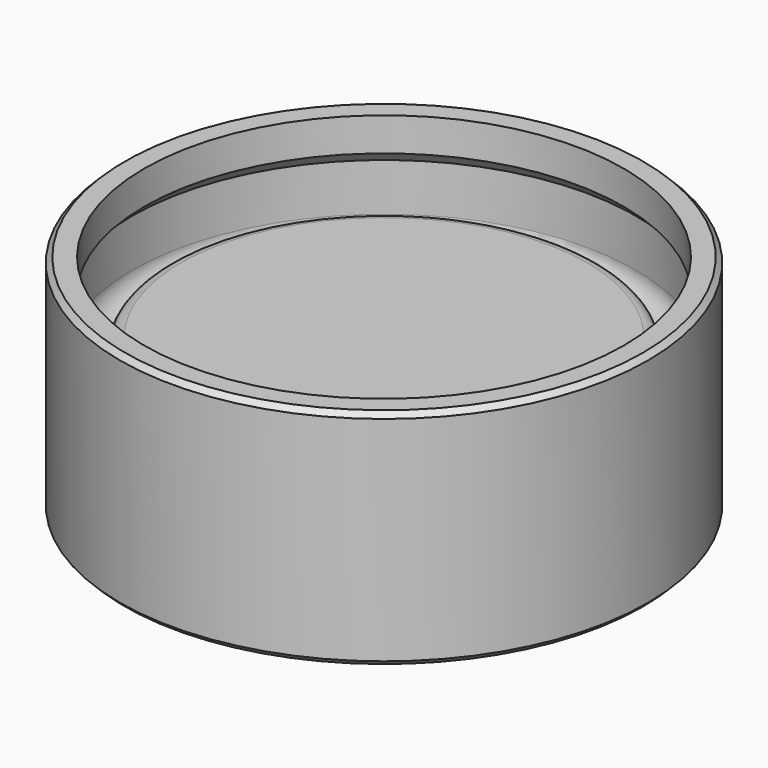
from build123d import *

# Parameters (mm, degrees)
F0_R            = 26
F1_DEPTH        = 22
F2_W            = 8.4
F2_H            = 2.4
F3_DEPTH        = 10
F3_COPIES_COUNT = 14
F4_R            = 4
F5_R            = 20
F6_DEPTH        = 13
F7_R            = 7.9
F8_DEPTH        = 1
F9_R            = 4.75
F10_DEPTH       = 0.8
F11_R           = 23.6
F12_DEPTH       = 7
F13_R           = 24.8
F13_R_2         = 21.2
F14_DEPTH       = 4
F14_DEPTH_BACK  = 4
F15_R           = 1.79999
F16_R           = 1.2
F17_S5_R        = 23.6
F17_T6_DEPTH    = 37
F18_R           = 1
F19_SIZE        = 0.5
F20_R           = 24.3
F21_DEPTH       = 1.5


# Not quite as in the source:
# - a fillet or chamfer that OpenCascade refuses, or shapes differently, is made with other operations: its cross-section is extruded or revolved along the edge and cut away or added
# - a fillet or chamfer is up to 0.001 mm smaller than in the source, because OpenCascade refuses the exact size
# - a pattern or mirror of a feature is missing from the dataset's text; its kind, count and spacing are read off the source's solid


with BuildPart() as f1:
    # F0 (on Top) → F1 (new body)
    with BuildSketch(Plane.XY):
        Circle(F0_R)
    extrude(amount=F1_DEPTH)

    # F2 (on face) → F3 (cut)
    with BuildSketch(Plane(origin=(0, 0, 0), x_dir=(1, 0, 0), z_dir=(0, 0, -1))):
        with Locations((0, 22)):
            Rectangle(F2_W, F2_H)
    f3 = extrude(amount=-F3_DEPTH, mode=Mode.SUBTRACT)

    # F3_copies: F3 ×14 about axis
    f3_copies_axis = Axis((0, 0, 0), (0, 0, 1))
    for i in range(1, F3_COPIES_COUNT):
        add(f3.rotate(f3_copies_axis, i * 360 / F3_COPIES_COUNT), mode=Mode.SUBTRACT)

    # F4
    f4_edges = [f1.edges().sort_by_distance(p)[0] for p in [
        (4.2, -22, 10),
        (-4.2, -22, 10),
        (-19.81895, -10.433083, 10),
        (-14.581635, -17.000468, 10),
        (-13.329512, -17.999003, 10),
        (-5.761373, -21.643627, 10),
        (-22.383002, -0.800763, 10),
        (-20.513826, -8.990158, 10),
        (5.761373, -21.643627, 10),
        (13.329512, -17.999003, 10),
        (14.581635, -17.000468, 10),
        (19.81895, -10.433083, 10),
        (20.513826, -8.990158, 10),
        (22.383002, -0.800763, 10),
        (-20.513826, 8.990158, 10),
        (-22.383002, 0.800763, 10),
        (-14.581635, 17.000468, 10),
        (-19.81895, 10.433083, 10),
        (-5.761373, 21.643627, 10),
        (-13.329512, 17.999003, 10),
        (22.383002, 0.800763, 10),
        (20.513826, 8.990158, 10),
        (4.2, 22, 10),
        (-4.2, 22, 10),
        (13.329512, 17.999003, 10),
        (5.761373, 21.643627, 10),
        (19.81895, 10.433083, 10),
        (14.581635, 17.000468, 10),
    ]]
    fillet(f4_edges, radius=F4_R)

    # F5 (on face) → F6 (cut)
    with BuildSketch(Plane(origin=(0, 0, 0), x_dir=(1, 0, 0), z_dir=(0, 0, -1))):
        Circle(F5_R)
    extrude(amount=-F6_DEPTH, mode=Mode.SUBTRACT)

    # F7 (on face) → F8 (cut)
    with BuildSketch(Plane(origin=(0, 0, 13), x_dir=(1, 0, 0), z_dir=(0, 0, -1))):
        Circle(F7_R)
    extrude(amount=-F8_DEPTH, mode=Mode.SUBTRACT)

    # F9 (on face) → F10 (join)
    with BuildSketch(Plane(origin=(0, 0, 14), x_dir=(1, 0, 0), z_dir=(0, 0, -1))):
        Circle(F9_R)
    extrude(amount=F10_DEPTH)

    # F11 (on face) → F12 (cut)
    with BuildSketch(Plane.XY.offset(22)):
        Circle(F11_R)
    extrude(amount=-F12_DEPTH, mode=Mode.SUBTRACT)

    # F13 (on face) → F14 (cut, two sides)
    with BuildSketch(Plane.XY.offset(15)) as f14_sk:
        Circle(F13_R)
        Circle(F13_R_2, mode=Mode.SUBTRACT)
    extrude(amount=-F14_DEPTH, mode=Mode.SUBTRACT)
    extrude(f14_sk.sketch, amount=F14_DEPTH_BACK, mode=Mode.SUBTRACT)

    # F15 (radius 1.8 in the source; OpenCascade refuses exactly that, so slightly less here)
    f15_edges = [f1.edges().sort_by_distance(p)[0] for p in [
        (-24.8, 0, 11),
        (-21.2, 0, 11),
    ]]
    fillet(f15_edges, radius=F15_R)

    # F16
    f16_edges = [f1.edges().sort_by_distance(p)[0] for p in [
        (-21.2, 0, 15),
    ]]
    fillet(f16_edges, radius=F16_R)

    # F17: chamfer of 1.5 on 1 edges, made by hand


with BuildPart() as f17_tool2:
    # F17_s3 → F17_t4 (revolve)
    with BuildSketch(Plane.XZ):
        Polygon((24.8, 17.5), (23.3, 19), (24.8, 19), align=None)
    revolve(axis=Axis((0, 0, 19), (0, 0, 1)))

    # F17_s5 → F17_t6 (cut, symmetric)
    with BuildSketch(Plane.XY.offset(18.2)):
        Circle(F17_S5_R)
    extrude(amount=F17_T6_DEPTH, both=True, mode=Mode.SUBTRACT)


with BuildPart() as f1_1:
    add(f1.part)

    # F17_t1: union F17_tool2
    add(f17_tool2.part)

    # F18
    f18_edges = [f1_1.edges().sort_by_distance(p)[0] for p in [
        (-20, 0, 13),
    ]]
    fillet(f18_edges, radius=F18_R)

    # F19
    f19_edges = [f1_1.edges().sort_by_distance(p)[0] for p in [
        (-26, 0, 0),
        (-26, 0, 22),
    ]]
    chamfer(f19_edges, length=F19_SIZE)

    # F20 (on face) → F21 (cut)
    with BuildSketch(Plane(origin=(0, 0, 0), x_dir=(1, 0, 0), z_dir=(0, 0, -1))):
        Circle(F20_R)
    extrude(amount=-F21_DEPTH, mode=Mode.SUBTRACT)


solid = f1_1.part
